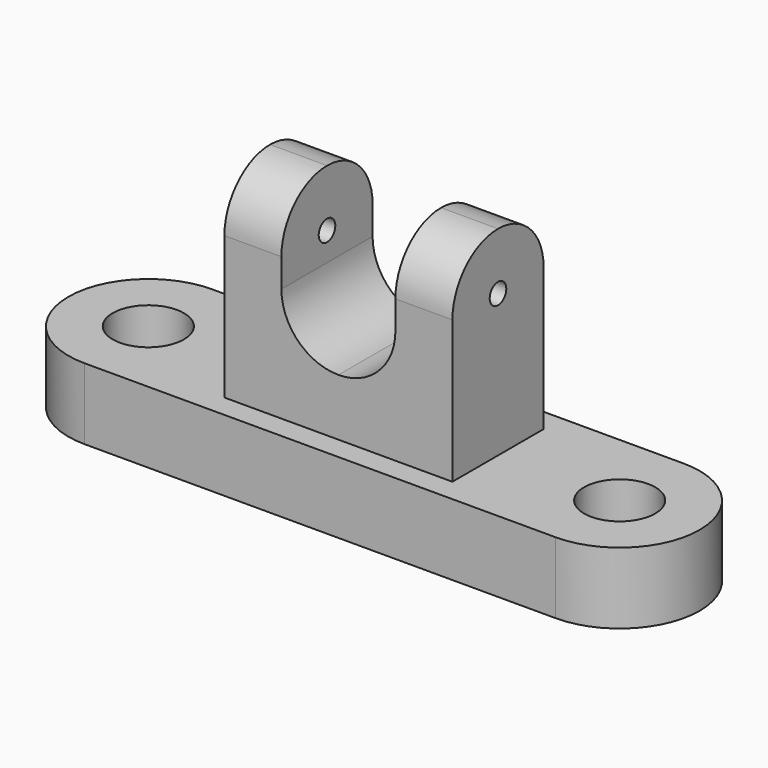
from build123d import *

# Parameters (mm, degrees)
F0_R     = 12.4944504689
F1_DEPTH = 25
F3_DEPTH = 20
F4_R     = 19.99999
F5_R     = 19.99999
F6_R     = 3.63588552
F7_DEPTH = 150.7420863042


# Not quite as in the source:
# - a fillet or chamfer is up to 0.001 mm smaller than in the source, because OpenCascade refuses the exact size


with BuildPart() as f1:
    # F0 (on Top) → F1 (new body)
    with BuildSketch(Plane.XY):
        with BuildLine():
            Line((-82.6911404729, -28.0499458313), (82.6911404729, -28.0499458313))
            ThreePointArc((82.6911404729, -28.0499458313), (110.7410863042, 0), (82.6911404729, 28.0499458313))
            Line((82.6911404729, 28.0499458313), (-82.6911404729, 28.0499458313))
            ThreePointArc((-82.6911404729, 28.0499458313), (-110.7410863042, 0), (-82.6911404729, -28.0499458313))
        make_face()
        with Locations((-82.6911404729, 0)):
            Circle(F0_R, mode=Mode.SUBTRACT)
        with Locations((82.6911404729, 0)):
            Circle(F0_R, mode=Mode.SUBTRACT)
    extrude(amount=F1_DEPTH)

    # F2 (on Front) → F3 (join, symmetric)
    with BuildSketch(Plane.XZ):
        Polygon((-40, 25), (40, 25), (40, 95), (20, 95), (20, 45), (-20, 45), (-20, 95), (-40, 95), align=None)
    extrude(amount=F3_DEPTH, both=True)

    # F4 (radius 20 in the source; OpenCascade refuses exactly that, so slightly less here)
    f4_edges = [f1.edges().sort_by_distance(p)[0] for p in [
        (-20, 0, 45),
        (20, 0, 45),
    ]]
    fillet(f4_edges, radius=F4_R)

    # F5 (radius 20 in the source; OpenCascade refuses exactly that, so slightly less here)
    f5_edges = [f1.edges().sort_by_distance(p)[0] for p in [
        (-30, -20, 95),
        (-30, 20, 95),
        (30, -20, 95),
        (30, 20, 95),
    ]]
    fillet(f5_edges, radius=F5_R)

    # F6 (on face) → F7 (cut, through all)
    with BuildSketch(Plane.YZ.offset(40)):
        with Locations((0, 75)):
            Circle(F6_R)
    extrude(amount=-F7_DEPTH, mode=Mode.SUBTRACT)


solid = f1.part
